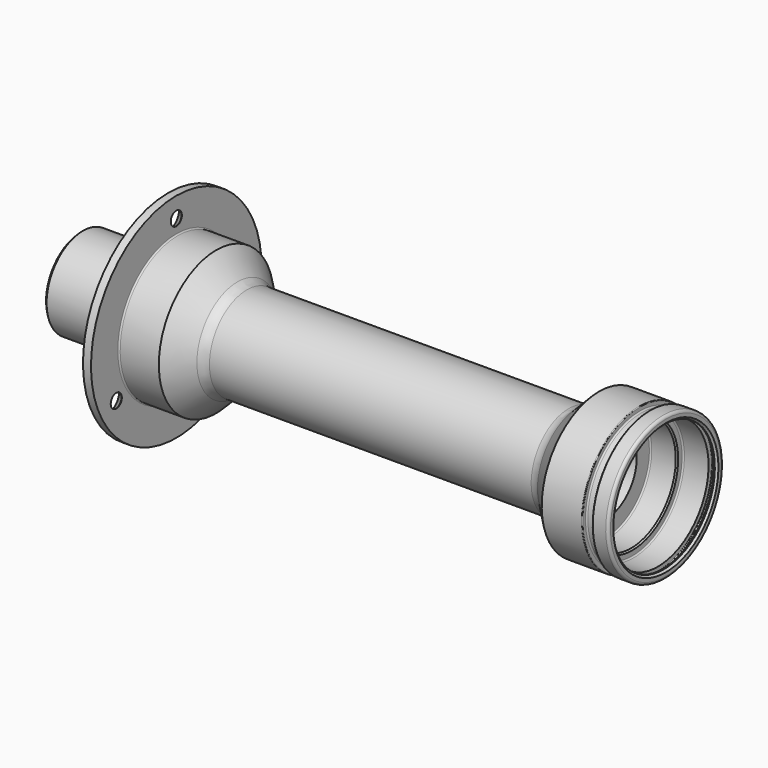
from build123d import *

# Parameters (mm, degrees)
F3_D           = 5.2
F3_DEPTH       = 100
F3_CSINK_D     = 10.2
F3_CSINK_ANGLE = 82
F3_TIP         = 1.5622376095
F4_R           = 5
F5_R           = 0.5
F6_R           = 2
F7_SIZE        = 1
F8_SIZE        = 0.75
F9_R           = 0.2
F10_R          = 0.5
F11_R          = 0.5
F12_SIZE       = 0.5
F13_R          = 0.25
F14_R          = 0.5
F15_R          = 1


with BuildPart() as f1:
    # F0 (on Front) → F1 (revolve)
    with BuildSketch(Plane.XZ):
        Polygon((-33.05, 14.55), (164.05, 14.55), (164.05, 20.9625), (174.05, 20.9625), (174.05, 23.7825), (183.6, 23.7825), (183.6, 25.5), (185.45, 25.5), (185.45, 23.9), (186.6, 23.9), (186.6, 26.95), (180.6, 26.95), (180.6, 24.95), (176.8, 24.95), (176.8, 26.95), (161.6, 26.95), (152.2, 17.55), (27.4, 17.55), (18, 26.95), (3, 26.95), (3, 40), (0, 40), (0, 22.8), (0, 17), (-33.05, 17), align=None)
    revolve(axis=Axis((35.5394743383, 0, 0), (1, 0, 0)))

    # F3
    with Locations(Plane(origin=(0, 0, 0), x_dir=(0, -1, 0), z_dir=(-1, 0, 0))):
        with Locations((-28.145825623, -16.25), (28.145825623, -16.25), (0, 32.5)):
            CounterSinkHole(F3_D / 2, F3_CSINK_D / 2, depth=F3_DEPTH, counter_sink_angle=F3_CSINK_ANGLE)
            with Locations((0, 0, -(F3_DEPTH + F3_TIP / 2))):  # 118° drill point
                Cone(0, F3_D / 2, F3_TIP, mode=Mode.SUBTRACT)

    # F4
    f4_edges = [f1.edges().sort_by_distance(p)[0] for p in [
        (27.4, 0, -17.55),
        (152.2, 0, -17.55),
    ]]
    fillet(f4_edges, radius=F4_R)

    # F5
    f5_edges = [f1.edges().sort_by_distance(p)[0] for p in [
        (3, 0, -26.95),
    ]]
    fillet(f5_edges, radius=F5_R)

    # F6
    f6_edges = [f1.edges().sort_by_distance(p)[0] for p in [
        (0, 0, -17),
    ]]
    fillet(f6_edges, radius=F6_R)

    # F7
    f7_edges = [f1.edges().sort_by_distance(p)[0] for p in [
        (-33.05, 0, -17),
        (-33.05, 0, -14.55),
    ]]
    chamfer(f7_edges, length=F7_SIZE)

    # F8
    f8_edges = [f1.edges().sort_by_distance(p)[0] for p in [
        (186.6, 0, -23.9),
    ]]
    chamfer(f8_edges, length=F8_SIZE)

    # F9
    f9_edges = [f1.edges().sort_by_distance(p)[0] for p in [
        (183.6, 0, -25.5),
        (185.45, 0, -25.5),
    ]]
    fillet(f9_edges, radius=F9_R)

    # F10
    f10_edges = [f1.edges().sort_by_distance(p)[0] for p in [
        (174.05, 0, -23.7825),
    ]]
    fillet(f10_edges, radius=F10_R)

    # F11
    f11_edges = [f1.edges().sort_by_distance(p)[0] for p in [
        (164.05, 0, -20.9625),
    ]]
    fillet(f11_edges, radius=F11_R)

    # F12
    f12_edges = [f1.edges().sort_by_distance(p)[0] for p in [
        (174.05, 0, -20.9625),
    ]]
    chamfer(f12_edges, length=F12_SIZE)

    # F13
    f13_edges = [f1.edges().sort_by_distance(p)[0] for p in [
        (176.8, 0, -26.95),
        (180.6, 0, -26.95),
    ]]
    fillet(f13_edges, radius=F13_R)

    # F14
    f14_edges = [f1.edges().sort_by_distance(p)[0] for p in [
        (176.8, 0, -24.95),
        (180.6, 0, -24.95),
    ]]
    fillet(f14_edges, radius=F14_R)

    # F15
    f15_edges = [f1.edges().sort_by_distance(p)[0] for p in [
        (186.6, 0, -26.95),
    ]]
    fillet(f15_edges, radius=F15_R)


solid = f1.part
